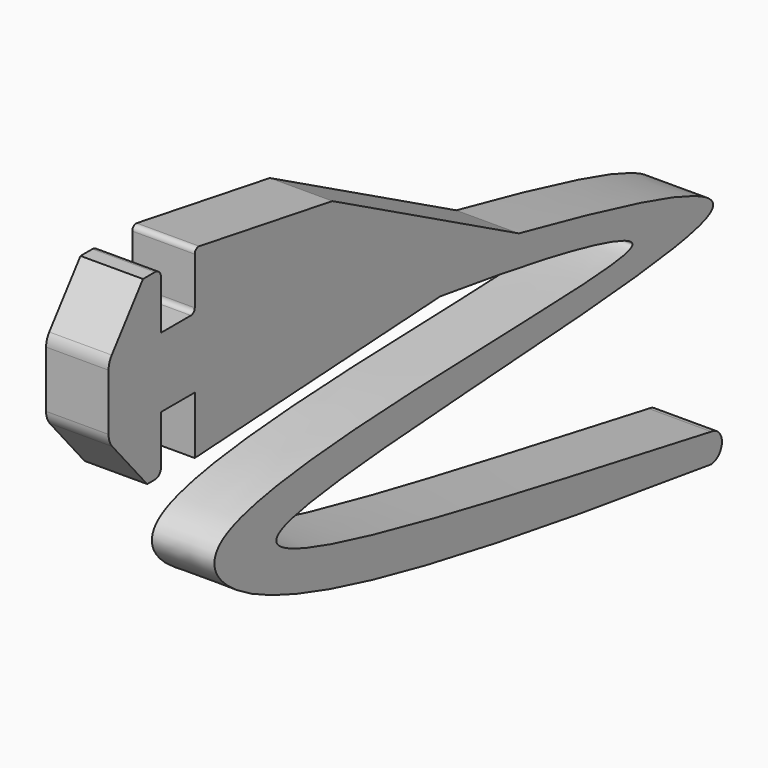
from build123d import *

# Parameters (mm, degrees)
F1_DEPTH = 6.5
F2_R     = 0.5


with BuildPart() as f1:
    # F0 (on Right) → F1 (new body)
    with BuildSketch(Plane.YZ):
        with BuildLine():
            Line((-2.3261857192, 7.8231747373), (-2.3261857192, 1.8231747373))
            Line((-2.3261857192, 1.8231747373), (-6.7077510927, 1.8231747373))
            Line((-6.7077510927, 1.8231747373), (-6.7077510927, 6.8951029659))
            ThreePointArc((-6.7077510927, 6.8951029659), (-6.9420656678, 7.4607883909), (-7.5077510927, 7.6951029659))
            Line((-7.5077510927, 7.6951029659), (-9.0546131166, 7.6951029659))
            Line((-9.0546131166, 7.6951029659), (-13.1169929958, 2.3829442588))
            ThreePointArc((-13.1169929958, 2.3829442588), (-13.4226828722, 1.8093478454), (-13.5282976587, 1.1680174602))
            Line((-13.5282976587, 1.1680174602), (-13.5282976587, -4.714347789))
            ThreePointArc((-13.5282976587, -4.714347789), (-13.4038536617, -5.40881858), (-13.0460079791, -6.01686665))
            Line((-13.0460079791, -6.01686665), (-8.5077510927, -11.3048970341))
            Line((-8.5077510927, -11.3048970341), (-7.5077510927, -11.3048970341))
            ThreePointArc((-7.5077510927, -11.3048970341), (-6.9420656678, -11.070582459), (-6.7077510927, -10.5048970341))
            Line((-6.7077510927, -10.5048970341), (-6.7077510927, -5.4329688054))
            Line((-6.7077510927, -5.4329688054), (-2.3261857192, -5.4329688054))
            add(Edge.make_bspline(
                [(29.5967873893, -9.603761956), (19.9915875977, -8.2575789777), (8.8285316572, -6.9078858502), (-2.3261857192, -5.4329688054)],
                knots=[0.854717852, 0.854717852, 0.854717852, 0.854717852, 1, 1, 1, 1], degree=3))
            add(Edge.make_bspline(
                [(64.8109703191, -39.3010818437), (37.7093056162, -35.6094605608), (2.9928587329, -30.3297260774), (-3.3768708565, -15.2714692161), (63.2058288641, -17.5013760989), (49.4841345426, -12.6487868731), (37.7129114005, -10.741248758), (29.5967873893, -9.603761956)],
                knots=[0, 0, 0, 0, 0.2956750024, 0.3797452222, 0.6483988176, 0.731958518, 0.854717852, 0.854717852, 0.854717852, 0.854717852], degree=3))
            ThreePointArc((64.8109703191, -39.3010818437), (66.206283861, -37.8047393877), (64.8109703191, -36.3083969317))
            add(Edge.make_bspline(
                [(39.8057358281, -7.9922291512), (56.820708357, -11.5700774026), (85.8899906987, -19.167635592), (-27.804311403, -20.0315678799), (33.7854768957, -30.6820395077), (64.8109703191, -36.3083969317)],
                knots=[0.1171792834, 0.1171792834, 0.1171792834, 0.1171792834, 0.3345486768, 0.664370096, 1, 1, 1, 1], degree=3))
            Line((39.8057358281, -7.9922291512), (15.5565273017, 4.8231747373))
            Line((15.5565273017, 4.8231747373), (-2.3261857192, 7.8231747373))
        make_face()
        with BuildLine():
            Line((-2.3261857192, -11.4329688054), (29.5967873893, -9.603761956))
            add(Edge.make_bspline(
                [(29.5967873893, -9.603761956), (19.9915875977, -8.2575789777), (8.8285316572, -6.9078858502), (-2.3261857192, -5.4329688054)],
                knots=[0.854717852, 0.854717852, 0.854717852, 0.854717852, 1, 1, 1, 1], degree=3))
            Line((-2.3261857192, -5.4329688054), (-2.3261857192, -11.4329688054))
        make_face()
    extrude(amount=F1_DEPTH)

    # F2
    f2_edges = [f1.edges().sort_by_distance(p)[0] for p in [
        (3.25, -2.326186, 7.823175),
        (3.25, -2.326186, 1.823175),
    ]]
    fillet(f2_edges, radius=F2_R)


solid = f1.part
